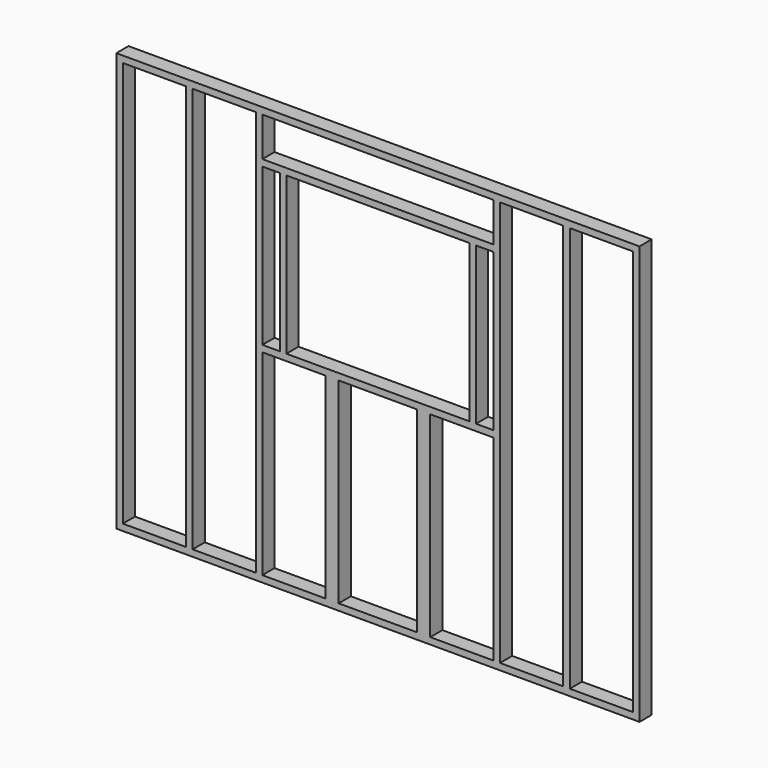
from build123d import *

# Parameters (mm, degrees)
F0_W     = 38.1
F0_H     = 2362.2
F0_H_2   = 1143
F0_H_3   = 914.4
F1_DEPTH = 88.9


# Not quite as in the source:
# - a feature names something its author has since deleted; it is built from what else it names


with BuildPart() as f1:
    # F0 (on Front) → F1 (new body)
    with BuildSketch(Plane.XZ):
        Polygon((1524, -1219.2), (1485.9, -1219.2), (1117.6, -1219.2), (1079.5, -1219.2), (711.2, -1219.2), (673.1, -1219.2), (304.8, -1219.2), (266.7, -1219.2), (228.6, -1219.2), (0, -1219.2), (-228.6, -1219.2), (-266.7, -1219.2), (-304.8, -1219.2), (-673.1, -1219.2), (-711.2, -1219.2), (-1079.5, -1219.2), (-1117.6, -1219.2), (-1485.9, -1219.2), (-1524, -1219.2), (-1524, -1257.3), (1524, -1257.3), align=None)
        with Locations((1504.95, -38.1)):
            Rectangle(F0_W, F0_H)
        with Locations((1098.55, -38.1)):
            Rectangle(F0_W, F0_H)
        Polygon((1117.6, 1143), (1485.9, 1143), (1524, 1143), (1524, 1181.1), (-1524, 1181.1), (-1524, 1143), (-1485.9, 1143), (-1117.6, 1143), (-1079.5, 1143), (-711.2, 1143), (-673.1, 1143), (673.1, 1143), (711.2, 1143), (1079.5, 1143), align=None)
        Polygon((673.1, -1219.2), (711.2, -1219.2), (711.2, 1143), (673.1, 1143), (673.1, 914.4), (673.1, 876.3), (673.1, -38.1), (673.1, -76.2), align=None)
        with Locations((-1504.95, -38.1)):
            Rectangle(F0_W, F0_H)
        with Locations((285.75, -647.7)):
            Rectangle(F0_W, F0_H_2)
        Polygon((304.8, -76.2), (673.1, -76.2), (673.1, -38.1), (571.5, -38.1), (533.4, -38.1), (-533.4, -38.1), (-571.5, -38.1), (-673.1, -38.1), (-673.1, -76.2), (-304.8, -76.2), (-266.7, -76.2), (-228.6, -76.2), (228.6, -76.2), (266.7, -76.2), align=None)
        with Locations((247.65, -647.7)):
            Rectangle(F0_W, F0_H_2)
        Polygon((673.1, 876.3), (673.1, 914.4), (-673.1, 914.4), (-673.1, 876.3), (-571.5, 876.3), (-533.4, 876.3), (533.4, 876.3), (571.5, 876.3), align=None)
        Polygon((-673.1, 914.4), (-673.1, 1143), (-711.2, 1143), (-711.2, -1219.2), (-673.1, -1219.2), (-673.1, -76.2), (-673.1, -38.1), (-673.1, 876.3), align=None)
        with Locations((-1098.55, -38.1)):
            Rectangle(F0_W, F0_H)
        with Locations((552.45, 419.1)):
            Rectangle(F0_W, F0_H_3)
        with Locations((-247.65, -647.7)):
            Rectangle(F0_W, F0_H_2)
        with Locations((-552.45, 419.1)):
            Rectangle(F0_W, F0_H_3)
        with Locations((-285.75, -647.7)):
            Rectangle(F0_W, F0_H_2)
    extrude(amount=F1_DEPTH)


solid = f1.part
